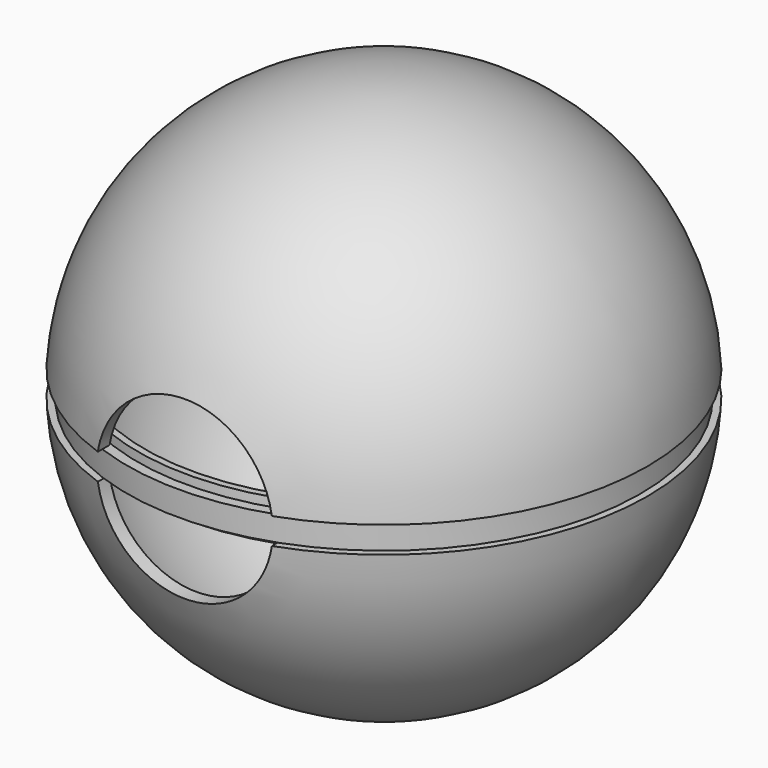
from build123d import *

# Parameters (mm, degrees)
F3_W      = 91.5835574269
F3_H      = 84.7303681076
F4_DEPTH  = 0.25
F2_R      = 12.7
F5_DEPTH  = 65.532
F8_R      = 1
F9_DEPTH  = 10
F10_R     = 1
F11_DEPTH = 5
F12_R     = 3.5
F12_R_2   = 1
F13_DEPTH = 5.5


with BuildPart() as f1:
    # F0 (on Front) → F1 (revolve)
    with BuildSketch(Plane.XZ):
        with BuildLine():
            Line((0, -36.1), (0, -38.1))
            ThreePointArc((0, -38.1), (26.2586128727, -27.6060727015), (38.0523451971, -1.905))
            Line((38.0523451971, -1.905), (36.0497014551, -1.905))
            ThreePointArc((36.0497014551, -1.905), (24.8439077039, -26.1914155784), (0, -36.1))
        make_face()
    revolve(axis=Axis((0, 0, 37.1), (0, 0, -1)))

    # F3 (on Top) → F4 (cut, symmetric)
    with BuildSketch(Plane.XY):
        with Locations((-0.697106123, -1.4025885612)):
            Rectangle(F3_W, F3_H)
    extrude(amount=F4_DEPTH, both=True, mode=Mode.SUBTRACT)


with BuildPart() as f1b:
    # F0 (on Front) → F1, piece 2 (revolve)
    with BuildSketch(Plane.XZ):
        with BuildLine():
            ThreePointArc((38.0523451971, 1.905), (26.2586128727, 27.6060727015), (0, 38.1))
            Line((0, 38.1), (0, 36.1))
            ThreePointArc((0, 36.1), (24.8439077039, 26.1914155784), (36.0497014551, 1.905))
            Line((36.0497014551, 1.905), (38.0523451971, 1.905))
        make_face()
    revolve(axis=Axis((0, 0, 37.1), (0, 0, -1)))


with BuildPart() as f5_tool:
    # F2 (on Front) → F5 (new body)
    with BuildSketch(Plane.XZ):
        Circle(F2_R)
    extrude(amount=F5_DEPTH)


with BuildPart() as f1_1:
    add(f1.part)

    # F5: cut by f5_tool
    add(f5_tool.part, mode=Mode.SUBTRACT)


with BuildPart() as f1b_1:
    add(f1b.part)

    # F5: cut by f5_tool
    add(f5_tool.part, mode=Mode.SUBTRACT)

    # F10 (on Right) → F11 (join, symmetric)
    with BuildSketch(Plane.YZ):
        with BuildLine():
            ThreePointArc((38.0523451971, 1.905), (38.0609207069, 1.7251999722), (38.0686466535, 1.5453614359))
            ThreePointArc((38.0686466535, 1.5453614359), (40.8398975537, -2.9933327526), (42.983035325, 1.873548896))
            Line((42.983035325, 1.873548896), (34.3259377148, 12.7))
            ThreePointArc((34.3259377148, 12.7), (35.8468471037, 7.3867146095), (36.5503895328, 1.905))
            Line((36.5503895328, 1.905), (38.0523451971, 1.905))
        make_face()
        with Locations((40.64, 0)):
            Circle(F10_R, mode=Mode.SUBTRACT)
    extrude(amount=F11_DEPTH, both=True)


with BuildPart() as f7:
    # F6 (on Front) → F7 (revolve)
    with BuildSketch(Plane.XZ):
        with BuildLine():
            Line((37.0523451971, -1.905), (37.0523451971, 1.655))
            Line((37.0523451971, 1.655), (35.5615097402, 1.655))
            ThreePointArc((35.5615097402, 1.655), (35.5268910919, 2.2803528997), (35.4812764004, 2.905))
            Line((35.4812764004, 2.905), (34.4812764004, 2.905))
            Line((34.4812764004, 2.905), (34.4812764004, -2.905))
            Line((34.4812764004, -2.905), (35.4812764004, -2.905))
            ThreePointArc((35.4812764004, -2.905), (35.5186546561, -2.4052383289), (35.5489940083, -1.905))
            Line((35.5489940083, -1.905), (37.0523451971, -1.905))
        make_face()
    revolve(axis=Axis((0, 0, -9.3113686889), (0, 0, -1)))

    # F8 (on Right) → F9 (join, symmetric)
    with BuildSketch(Plane.YZ):
        with BuildLine():
            Line((35.0969918072, -1.905), (38.3224635925, -1.905))
            ThreePointArc((38.3224635925, -1.905), (43.6359723613, 0.1554014481), (38.1378059628, 1.655))
            Line((38.1378059628, 1.655), (35.0969918072, 1.655))
            Line((35.0969918072, 1.655), (35.0969918072, -1.905))
        make_face()
        with Locations((40.64, 0)):
            Circle(F8_R, mode=Mode.SUBTRACT)
    extrude(amount=F9_DEPTH, both=True)

    # F12 (on Right) → F13 (cut, symmetric)
    with BuildSketch(Plane.YZ):
        with Locations((40.64, 0)):
            Circle(F12_R)
        with Locations((40.64, 0)):
            Circle(F12_R_2, mode=Mode.SUBTRACT)
    extrude(amount=F13_DEPTH, both=True, mode=Mode.SUBTRACT)


solid = Compound([f1_1.part, f1b_1.part, f7.part])
